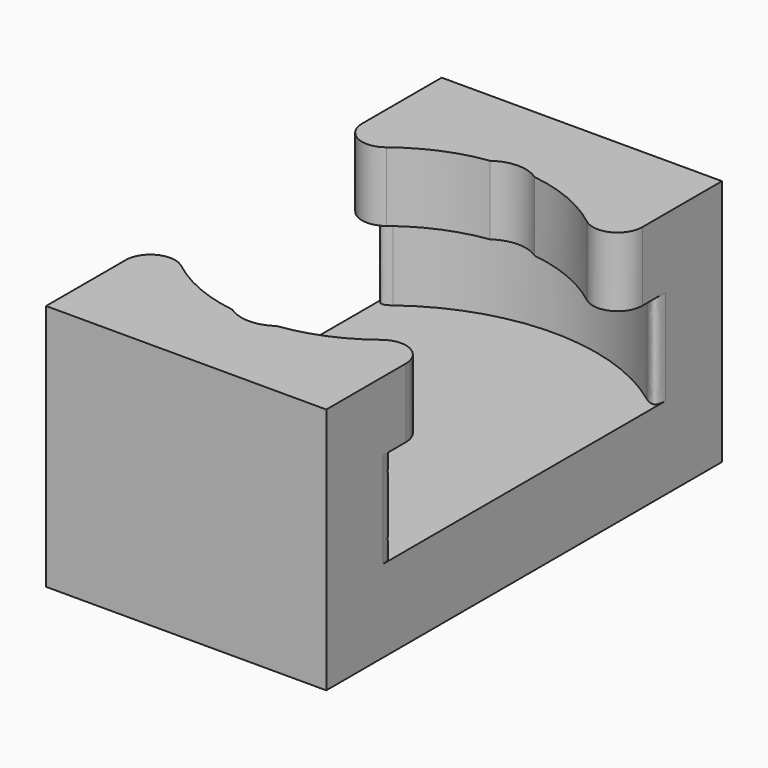
from build123d import *

# Parameters (mm, degrees)
F0_R         = 12.875
F1_DEPTH     = 5.8
F2_R         = 9.875
F3_DEPTH     = 12
F5_DEPTH     = 5
F7_W         = 30
F7_H         = 30
F7_W_2       = 18
F7_H_2       = 27
F8_DEPTH     = 10
F15_W        = 17
F15_H        = 30
F16_DEPTH    = 15
F18_R        = 1.5
F19_T1_DEPTH = 5.8


# Not quite as in the source:
# - a fillet or chamfer that OpenCascade refuses, or shapes differently, is made with other operations: its cross-section is extruded or revolved along the edge and cut away or added
# - a feature names something its author has since deleted; it is built from what else it names


with BuildPart() as f1:
    # F0 (on Top) → F1 (new body)
    with BuildSketch(Plane.XY):
        Circle(F0_R)
    extrude(amount=-F1_DEPTH)

    # F2 (on Top) → F3 (join)
    with BuildSketch(Plane.XY):
        Circle(F2_R)
    extrude(amount=F3_DEPTH)


with BuildPart() as f5:
    # F4 (on Top) → F5 (new body)
    with BuildSketch(Plane.XY):
        with BuildLine():
            ThreePointArc((-2.19192449, 8.7487287819), (-0.0332522533, 9.0190732649), (2.1273547272, 8.7646534521))
            ThreePointArc((2.1273547272, 8.7646534521), (-0.0376344683, 10.2076699565), (-2.19192449, 8.7487287819))
        make_face()
    extrude(amount=F5_DEPTH)


with BuildPart() as f6_1:
    # F6: instance of F5
    add(f5.part.mirror(Plane.XZ))


with BuildPart() as f8:
    # F7 (on Top) → F8 (new body, symmetric)
    with BuildSketch(Plane.XY):
        Rectangle(F7_W, F7_H)
        Rectangle(F7_W_2, F7_H_2, mode=Mode.SUBTRACT)
    extrude(amount=F8_DEPTH, both=True)


with BuildPart() as f1_1:
    add(f1.part)

    # F9: cut F8
    add(f8.part, mode=Mode.SUBTRACT)


with BuildPart() as f16:
    # F15 (on face) → F16 (new body)
    with BuildSketch(Plane(origin=(0, 0, -10.8), x_dir=(1, 0, 0), z_dir=(0, 0, -1))):
        Rectangle(F15_W, F15_H)
    extrude(amount=-F16_DEPTH)

    # F17: cut F6_1, F5, F1
    add(f6_1.part, mode=Mode.SUBTRACT)
    add(f5.part, mode=Mode.SUBTRACT)
    add(f1_1.part, mode=Mode.SUBTRACT)

    # F18
    f18_edges = [f16.edges().sort_by_distance(p)[0] for p in [
        (8.5, -5.026492, 2.1),
        (8.5, 5.026492, 2.1),
        (-8.5, 5.026492, 2.1),
        (-8.5, -5.026492, 2.1),
    ]]
    fillet(f18_edges, radius=F18_R)

    # F19: fillet of radius 0.5 on 4 edges, made by hand

    # F19_s2 → F19_t1 (cut)
    with BuildSketch(Plane.XY.offset(-5.8)):
        with BuildLine():
            add(Edge.make_bspline(
                [(-7.7009345794, 10.3180052143), (-8.5, 9.7216156603), (-8.5, 10.718704446)],
                knots=[0, 0, 0, 1, 1, 1], degree=2, weights=[1, 1, 1]))
            Line((-8.5, 10.718704446), (-8.5, 9.6703477187))
            ThreePointArc((-8.5, 9.6703477187), (-8.106937484, 10.0021592484), (-7.7009345794, 10.3180052143))
        make_face()
        with BuildLine():
            add(Edge.make_bspline(
                [(-7.7009345794, -10.3180052143), (-8.5, -9.7216156603), (-8.5, -10.718704446)],
                knots=[0, 0, 0, 1, 1, 1], degree=2, weights=[1, 1, 1]))
            Line((-8.5, -10.718704446), (-8.5, -9.6703477187))
            ThreePointArc((-8.5, -9.6703477187), (-8.106937484, -10.0021592484), (-7.7009345794, -10.3180052143))
        make_face()
        with BuildLine():
            add(Edge.make_bspline(
                [(8.5, 10.718704446), (8.5, 9.7216156603), (7.7009345794, 10.3180052143)],
                knots=[0, 0, 0, 1, 1, 1], degree=2, weights=[1, 1, 1]))
            ThreePointArc((7.7009345794, 10.3180052143), (8.106937484, 10.0021592484), (8.5, 9.6703477187))
            Line((8.5, 9.6703477187), (8.5, 10.718704446))
        make_face()
        with BuildLine():
            add(Edge.make_bspline(
                [(8.5, -10.718704446), (8.5, -9.7216156603), (7.7009345794, -10.3180052143)],
                knots=[0, 0, 0, 1, 1, 1], degree=2, weights=[1, 1, 1]))
            ThreePointArc((7.7009345794, -10.3180052143), (8.106937484, -10.0021592484), (8.5, -9.6703477187))
            Line((8.5, -9.6703477187), (8.5, -10.718704446))
        make_face()
    extrude(amount=F19_T1_DEPTH, mode=Mode.SUBTRACT)


solid = f16.part
